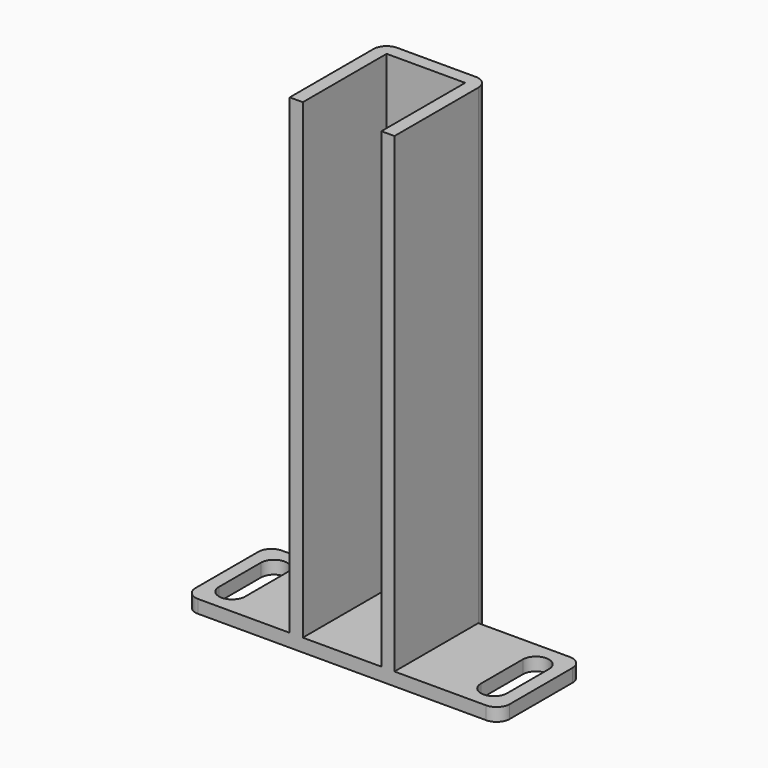
from build123d import *

# Parameters (mm, degrees)
F1_DEPTH = 3.175
F2_W     = 3.175
F2_H     = 25.4
F3_DEPTH = 114.3
F4_W     = 3.175
F4_H     = 114.3
F4_W_2   = 19.05
F4_H_2   = 3.175
F5_DEPTH = 3.175
F6_D     = 6.35
F7_R     = 3.17499


# Not quite as in the source:
# - a fillet or chamfer is up to 0.001 mm smaller than in the source, because OpenCascade refuses the exact size


with BuildPart() as f1:
    # F0 (on Top) → F1 (new body)
    with BuildSketch(Plane.XY):
        with BuildLine():
            Line((34.925, 12.7), (-34.925, 12.7))
            ThreePointArc((-34.925, 12.7), (-37.1700640303, 11.7700640303), (-38.1, 9.525))
            Line((-38.1, 9.525), (-38.1, -9.525))
            ThreePointArc((-38.1, -9.525), (-37.1700640303, -11.7700640303), (-34.925, -12.7))
            Line((-34.925, -12.7), (34.925, -12.7))
            ThreePointArc((34.925, -12.7), (37.1700640303, -11.7700640303), (38.1, -9.525))
            Line((38.1, -9.525), (38.1, 9.525))
            ThreePointArc((38.1, 9.525), (37.1700640303, 11.7700640303), (34.925, 12.7))
        make_face()
        with BuildLine():
            Line((-34.925, -6.35), (-34.925, 6.35))
            ThreePointArc((-34.925, 6.35), (-31.75, 9.525), (-28.575, 6.35))
            Line((-28.575, 6.35), (-28.575, -6.35))
            ThreePointArc((-28.575, -6.35), (-31.75, -9.525), (-34.925, -6.35))
        make_face(mode=Mode.SUBTRACT)
        with BuildLine():
            Line((28.575, -6.35), (28.575, 6.35))
            ThreePointArc((28.575, 6.35), (31.75, 9.525), (34.925, 6.35))
            Line((34.925, 6.35), (34.925, -6.35))
            ThreePointArc((34.925, -6.35), (31.75, -9.525), (28.575, -6.35))
        make_face(mode=Mode.SUBTRACT)
    extrude(amount=F1_DEPTH)

    # F2 (on face) → F3 (join)
    with BuildSketch(Plane.XY.offset(3.175)):
        with Locations((11.1125, 0)):
            Rectangle(F2_W, F2_H)
        with Locations((-11.1125, 0)):
            Rectangle(F2_W, F2_H)
    extrude(amount=F3_DEPTH)

    # F4 (on face) → F5 (join)
    with BuildSketch(Plane(origin=(0, 12.7, 0), x_dir=(-1, 0, 0), z_dir=(0, 1, 0))):
        with Locations((-11.1125, 60.325)):
            Rectangle(F4_W, F4_H)
        with Locations((0, 60.325)):
            Rectangle(F4_W_2, F4_H)
        with Locations((11.1125, 60.325)):
            Rectangle(F4_W, F4_H)
        with Locations((0, 1.5875)):
            Rectangle(F4_W_2, F4_H_2)
        with Locations((-11.1125, 1.5875)):
            Rectangle(F4_W, F4_H_2)
        with Locations((11.1125, 1.5875)):
            Rectangle(F4_W, F4_H_2)
    extrude(amount=F5_DEPTH)

    # F6 (through all)
    with Locations(Plane(origin=(0, 12.7, 0), x_dir=(-1, 0, 0), z_dir=(0, -1, 0))):
        with Locations((0, -28.575), (0, -60.325), (0, -92.075)):
            Hole(F6_D / 2)

    # F7 (radius 3.175 in the source; OpenCascade refuses exactly that, so slightly less here)
    f7_edges = [f1.edges().sort_by_distance(p)[0] for p in [
        (0, 15.875, 0),
        (12.7, 15.875, 58.7375),
        (-12.7, 15.875, 58.7375),
    ]]
    fillet(f7_edges, radius=F7_R)


solid = f1.part
